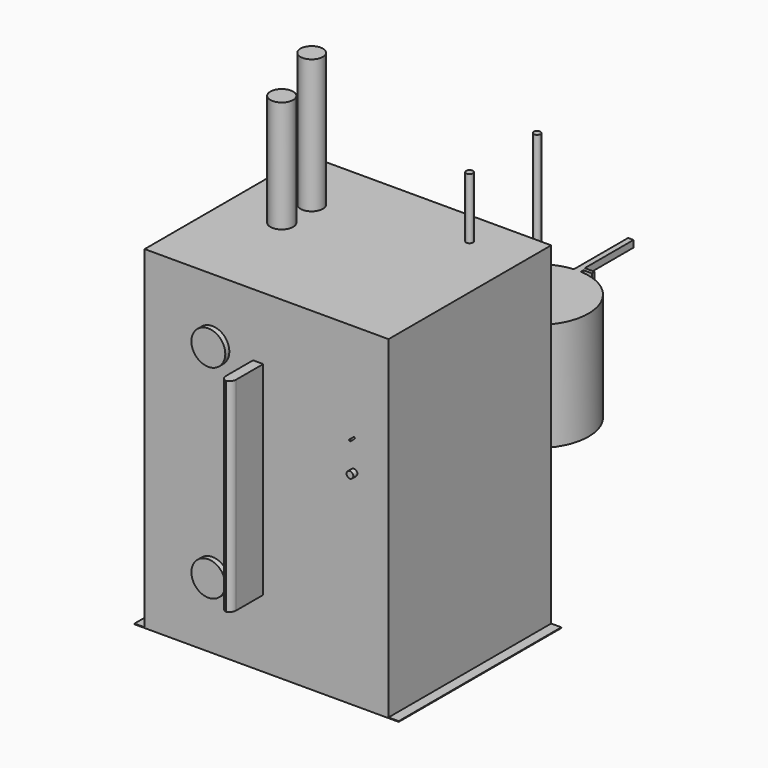
from build123d import *

# Parameters (mm, degrees)
F0_W         = 457.2
F0_H         = 381
F1_DEPTH     = 625.475
F2_R         = 21.0935486288
F3_DEPTH     = 250.825
F4_R         = 21.4047690014
F5_DEPTH     = 209.55
F6_R         = 31.75
F6_R_2       = 1.5875
F6_R_3       = 6.35
F7_DEPTH     = 9.525
F8_W         = 19.05
F8_H         = 381
F9_DEPTH     = 76.2
F10_T1_DEPTH = 444.5
F12_R        = 96.52
F13_DEPTH    = 203.2
F15_DEPTH    = 12.7
F16_R        = 6.35
F17_DEPTH    = 266.7
F18_R        = 6.35
F19_DEPTH    = 114.3
F20_R        = 9.525
F21_DEPTH    = 170.18
F22_W        = 381
F22_H        = 1.27
F23_DEPTH    = 19.05
F24_W        = 381
F24_H        = 1.27
F25_DEPTH    = 19.05
F28_DEPTH    = 3.175


# Not quite as in the source:
# - a fillet or chamfer that OpenCascade refuses, or shapes differently, is made with other operations: its cross-section is extruded or revolved along the edge and cut away or added


with BuildPart() as f1:
    # F0 (on Top) → F1 (new body)
    with BuildSketch(Plane.XY):
        Rectangle(F0_W, F0_H)
    extrude(amount=-F1_DEPTH)

    # F2 (on face) → F3 (join)
    with BuildSketch(Plane.XY):
        with Locations((-125.4702359438, 72.0090046525)):
            Circle(F2_R)
    extrude(amount=F3_DEPTH)

    # F4 (on face) → F5 (join)
    with BuildSketch(Plane.XY):
        with Locations((-124.0155026317, 0)):
            Circle(F4_R)
    extrude(amount=F5_DEPTH)

    # F6 (on face) → F7 (join)
    with BuildSketch(Plane.XZ.offset(190.5)):
        with Locations((-101.6, -117.475)):
            Circle(F6_R)
        with Locations((-101.6, -498.475)):
            Circle(F6_R)
        with Locations((163.7871414423, -184.2048317194)):
            Circle(F6_R_2)
        with Locations((163.7871414423, -241.1169111729)):
            Circle(F6_R_3)
    extrude(amount=F7_DEPTH)

    # F8 (on face) → F9 (join)
    with BuildSketch(Plane.XZ.offset(190.5)):
        with Locations((-15.875, -307.975)):
            Rectangle(F8_W, F8_H)
    extrude(amount=F9_DEPTH)

    # F10: fillet of radius 12.7 on 2 edges, made by hand

    # F10_s2 → F10_t1 (cut)
    with BuildSketch(Plane.XY.offset(-530.225)):
        with BuildLine():
            ThreePointArc((-25.4, -254), (-21.6802561211, -262.9802561211), (-12.7, -266.7))
            Line((-12.7, -266.7), (-25.4, -266.7))
            Line((-25.4, -266.7), (-25.4, -254))
        make_face()
        with BuildLine():
            ThreePointArc((-6.35, -254), (-10.0697438789, -262.9802561211), (-19.05, -266.7))
            Line((-19.05, -266.7), (-6.35, -266.7))
            Line((-6.35, -266.7), (-6.35, -254))
        make_face()
    extrude(amount=F10_T1_DEPTH, mode=Mode.SUBTRACT)

    # F12 (on offset) → F13 (join)
    with BuildSketch(Plane.XY.offset(-152.4)):
        with Locations((127.0715296268, 284.48)):
            Circle(F12_R)
    extrude(amount=-F13_DEPTH)

    # F14 (on face) → F15 (join)
    with BuildSketch(Plane.XY.offset(-152.4)):
        Polygon((119.0875349175, 393.3692209579), (119.0875349175, 380.6692209579), (131.7875349175, 380.8847182149), (131.7875349175, 387.0192209579), (147.6625349175, 387.0192209579), (147.6625349175, 393.3692209579), (129.2475349175, 393.3692209579), (129.2475349175, 507.6692209579), (119.0875349175, 507.6692209579), align=None)
    extrude(amount=-F15_DEPTH)

    # F16 (on face) → F17 (join)
    with BuildSketch(Plane.XY.offset(-152.4)):
        with Locations((127.0715296268, 284.48)):
            Circle(F16_R)
    extrude(amount=F17_DEPTH)

    # F18 (on face) → F19 (join)
    with BuildSketch(Plane.XY):
        with Locations((127.4323694774, 125.7402606834)):
            Circle(F18_R)
    extrude(amount=F19_DEPTH)

    # F20 (on Right) → F21 (join, symmetric)
    with BuildSketch(Plane.YZ):
        with Locations((197.485, -555.625)):
            Circle(F20_R)
    extrude(amount=F21_DEPTH, both=True)

    # F22 (on face) → F23 (join)
    with BuildSketch(Plane(origin=(-228.6, 0, 0), x_dir=(0, -1, 0), z_dir=(-1, 0, 0))):
        with Locations((0, -624.84)):
            Rectangle(F22_W, F22_H)
    extrude(amount=F23_DEPTH)

    # F24 (on face) → F25 (join)
    with BuildSketch(Plane.YZ.offset(228.6)):
        with Locations((0, -624.84)):
            Rectangle(F24_W, F24_H)
    extrude(amount=F25_DEPTH)

    # F27 (on offset) → F28 (join)
    with BuildSketch(Plane.XZ.offset(-205.74)):
        with BuildLine():
            Line((-127, -555.625), (-107.95, -555.625))
            Line((-107.95, -555.625), (-107.95, -460.375))
            ThreePointArc((-107.95, -460.375), (-109.8098719395, -455.8848719395), (-114.3, -454.025))
            Line((-114.3, -454.025), (-120.65, -454.025))
            ThreePointArc((-120.65, -454.025), (-125.1401280605, -455.8848719395), (-127, -460.375))
            Line((-127, -460.375), (-127, -555.625))
        make_face()
    extrude(amount=-F28_DEPTH)


solid = f1.part
